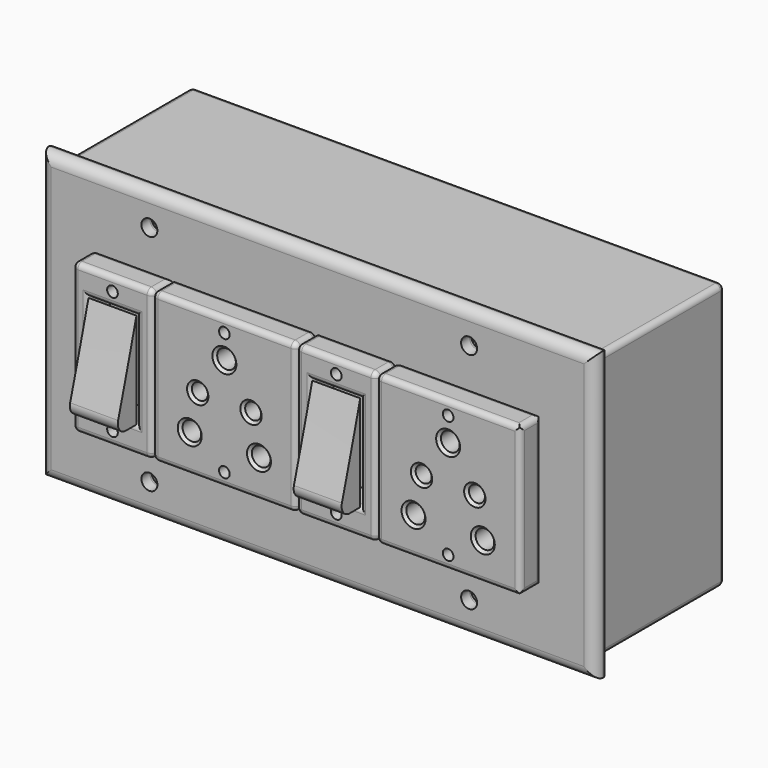
from build123d import *

# Parameters (mm, degrees)
F0_W           = 10
F0_H           = 5
F1_DEPTH       = 3
F2_T           = -0.5
F3_W           = 10.4
F3_H           = 5.4
F3_W_2         = 10
F3_H_2         = 5
F3_W_3         = 9
F3_H_3         = 4
F4_DEPTH       = 0.3
F5_W           = 1.5
F5_H           = 2.8
F5_W_2         = 0.9
F5_H_2         = 1.8
F6_DEPTH       = 0.5
F5_W_3         = 2.7
F5_R           = 0.175
F5_R_2         = 0.15
F7_DEPTH       = 0.5
F9_DEPTH       = 0.9
F10_R          = 0.1
F11_SIZE       = 0.05
F12_R          = 0.1
F13_R          = 0.2
F15_D          = 0.2
F15_DEPTH      = 0.5
F15_TIP        = 0.0600860619
F15_2_D        = 0.2
F15_2_DEPTH    = 0.5
F15_2_TIP      = 0.0600860619
F15_3_D        = 0.2
F15_3_DEPTH    = 0.5
F15_3_TIP      = 0.0600860619
F17_D          = 0.3
F17_DEPTH      = 0.5
F17_TIP        = 0.0901290929
F17_2_D        = 0.3
F17_2_DEPTH    = 0.5
F17_2_TIP      = 0.0901290929
F22_T1_DEPTH   = 2.6
F22_S5_W       = 0.1
F22_S5_H       = 0.1
F22_T6_DEPTH   = 0.1
F22_S11_W      = 0.1
F22_S11_H      = 0.1
F22_T12_DEPTH  = 0.1
F22_2_T1_DEPTH = 3.1
F23_R          = 0.09999
F23_2_R        = 0.09999


# Not quite as in the source:
# - a fillet or chamfer that OpenCascade refuses, or shapes differently, is made with other operations: its cross-section is extruded or revolved along the edge and cut away or added
# - a fillet or chamfer is up to 0.001 mm smaller than in the source, because OpenCascade refuses the exact size


with BuildPart() as f1:
    # F0 (on Front) → F1 (new body)
    with BuildSketch(Plane.XZ):
        Rectangle(F0_W, F0_H)
    extrude(amount=F1_DEPTH)

    # F2
    f2_openings = [f1.faces().sort_by_distance(p)[0] for p in [
        (0, -3, 0),
    ]]
    offset(amount=F2_T, openings=f2_openings)

    # F17
    with Locations(Plane.XZ.offset(3.3)):
        with Locations((-3.1569213606, 2.1), (2.8430786394, 2.1), (-3.1569213606, -2.1), (2.8430786394, -2.1)):
            Hole(F17_D / 2, depth=F17_DEPTH)
            with Locations((0, 0, -(F17_DEPTH + F17_TIP / 2))):  # 118° drill point
                Cone(0, F17_D / 2, F17_TIP, mode=Mode.SUBTRACT)

    # F23 (radius 0.1 in the source; OpenCascade refuses exactly that, so slightly less here)
    f23_edges = [f1.edges().sort_by_distance(p)[0] for p in [
        (5, -1.5, -2.5),
        (5, -1.5, 2.5),
        (5, 0, 0),
        (5, -3, 0),
        (-5, -1.5, 2.5),
        (0, 0, 2.5),
        (0, -3, 2.5),
        (0, 0, -2.5),
        (-5, 0, 0),
        (-5, -1.5, -2.5),
        (-5, -3, 0),
    ]]
    fillet(f23_edges, radius=F23_R)


with BuildPart() as f4:
    # F3 (on face) → F4 (new body)
    with BuildSketch(Plane.XZ.offset(3)):
        Rectangle(F3_W, F3_H)
        Rectangle(F3_W_2, F3_H_2, mode=Mode.SUBTRACT)
        Rectangle(F3_W_2, F3_H_2)
        Rectangle(F3_W_3, F3_H_3, mode=Mode.SUBTRACT)
        Rectangle(F3_W_3, F3_H_3)
    extrude(amount=F4_DEPTH)

    # F13
    f13_edges = [f4.edges().sort_by_distance(p)[0] for p in [
        (0, -3.3, -2.7),
        (5.2, -3.3, 0),
        (0, -3.3, 2.7),
        (-5.2, -3.3, 0),
    ]]
    fillet(f13_edges, radius=F13_R)

    # F15
    with Locations(Plane.XZ.offset(3.8)):
        with Locations((-3.45, 1.15), (-1.35, 1.15), (-3.45, -1.15), (-1.35, -1.15)):
            Hole(F15_D / 2, depth=F15_DEPTH)
            with Locations((0, 0, -(F15_DEPTH + F15_TIP / 2))):  # 118° drill point
                Cone(0, F15_D / 2, F15_TIP, mode=Mode.SUBTRACT)

    # F17#2
    with Locations(Plane.XZ.offset(3.3)):
        with Locations((-3.1569213606, 2.1), (2.8430786394, 2.1), (-3.1569213606, -2.1), (2.8430786394, -2.1)):
            Hole(F17_2_D / 2, depth=F17_2_DEPTH)
            with Locations((0, 0, -(F17_2_DEPTH + F17_2_TIP / 2))):  # 118° drill point
                Cone(0, F17_2_D / 2, F17_2_TIP, mode=Mode.SUBTRACT)

    # F23#2 (radius 0.1 in the source; OpenCascade refuses exactly that, so slightly less here)
    f23_2_edges = [f4.edges().sort_by_distance(p)[0] for p in [
        (0, -3, -2.7),
        (-5.2, -3, 0),
        (5.2, -3, 0),
        (0, -3, 2.7),
        (-3.306921, -3, -2.1),
        (2.693079, -3, -2.1),
        (-3.306921, -3, 2.1),
        (2.693079, -3, 2.1),
    ]]
    fillet(f23_2_edges, radius=F23_2_R)


with BuildPart() as f6:
    # F5 (on face) → F6 (new body)
    with BuildSketch(Plane.XZ.offset(3.3)):
        with Locations((-3.45, 0)):
            Rectangle(F5_W, F5_H)
        with Locations((-3.45, 0)):
            Rectangle(F5_W_2, F5_H_2, mode=Mode.SUBTRACT)
    extrude(amount=F6_DEPTH)

    # F10
    f10_edges = [f6.edges().sort_by_distance(p)[0] for p in [
        (-3.45, -3.8, -1.4),
        (-2.7, -3.8, 0),
        (-3.45, -3.8, 1.4),
        (-4.2, -3.8, 0),
        (-3, -3.8, 0),
        (-3.45, -3.8, -0.9),
        (-3.9, -3.8, 0),
        (-3.45, -3.8, 0.9),
        (-4.2, -3.55, 1.4),
        (-4.2, -3.55, -1.4),
        (-4.2, -3.3, 0),
        (-3.45, -3.3, 1.4),
        (-3.45, -3.3, -1.4),
        (-2.7, -3.55, 1.4),
        (-2.7, -3.55, -1.4),
    ]]
    fillet(f10_edges, radius=F10_R)

    # F15#2
    with Locations(Plane.XZ.offset(3.8)):
        with Locations((-3.45, 1.15), (-1.35, 1.15), (-3.45, -1.15), (-1.35, -1.15)):
            Hole(F15_2_D / 2, depth=F15_2_DEPTH)
            with Locations((0, 0, -(F15_2_DEPTH + F15_2_TIP / 2))):  # 118° drill point
                Cone(0, F15_2_D / 2, F15_2_TIP, mode=Mode.SUBTRACT)


with BuildPart() as f7:
    # F5 (on face) → F7 (new body)
    with BuildSketch(Plane.XZ.offset(3.3)):
        with Locations((-1.35, 0)):
            Rectangle(F5_W_3, F5_H)
        with Locations((-2, -0.7)):
            Circle(F5_R, mode=Mode.SUBTRACT)
        with Locations((-0.7, -0.7)):
            Circle(F5_R, mode=Mode.SUBTRACT)
        with Locations((-1.85, 0)):
            Circle(F5_R_2, mode=Mode.SUBTRACT)
        with Locations((-0.85, 0)):
            Circle(F5_R_2, mode=Mode.SUBTRACT)
        with Locations((-1.35, 0.7)):
            Circle(F5_R, mode=Mode.SUBTRACT)
    extrude(amount=F7_DEPTH)

    # F11
    f11_edges = [f7.edges().sort_by_distance(p)[0] for p in [
        (-1.525, -3.8, 0.7),
        (-2, -3.8, 0),
        (-1, -3.8, 0),
        (-2.175, -3.8, -0.7),
        (-0.875, -3.8, -0.7),
    ]]
    chamfer(f11_edges, length=F11_SIZE)

    # F12
    f12_edges = [f7.edges().sort_by_distance(p)[0] for p in [
        (0, -3.55, 1.4),
        (-2.7, -3.55, 1.4),
        (-1.35, -3.3, 1.4),
        (-1.35, -3.8, 1.4),
        (0, -3.55, -1.4),
        (0, -3.3, 0),
        (0, -3.8, 0),
        (-2.7, -3.55, -1.4),
        (-1.35, -3.3, -1.4),
        (-1.35, -3.8, -1.4),
    ]]
    fillet(f12_edges, radius=F12_R)

    # F15#3
    with Locations(Plane.XZ.offset(3.8)):
        with Locations((-3.45, 1.15), (-1.35, 1.15), (-3.45, -1.15), (-1.35, -1.15)):
            Hole(F15_3_D / 2, depth=F15_3_DEPTH)
            with Locations((0, 0, -(F15_3_DEPTH + F15_3_TIP / 2))):  # 118° drill point
                Cone(0, F15_3_D / 2, F15_3_TIP, mode=Mode.SUBTRACT)


with BuildPart() as f9:
    # F8 (on face) → F9 (new body, through all)
    with BuildSketch(Plane.YZ.offset(-3.9)):
        with BuildLine():
            Line((-4.0475652224, -0.9), (-3.8, -0.9))
            Line((-3.8, -0.9), (-3.8, 0.9))
            ThreePointArc((-3.8, 0.9), (-4.0115602658, 0.1201773265), (-4.230279809, -0.6576677157))
            ThreePointArc((-4.230279809, -0.6576677157), (-4.1993130034, -0.8243672998), (-4.0475652224, -0.9))
        make_face()
    extrude(amount=F9_DEPTH)


with BuildPart() as f19_1:
    # F19: instance of F6
    add(f6.part.mirror(Plane.YZ.offset(-1.35)))


with BuildPart() as f19_2:
    # F19: instance of F9
    add(f9.part.mirror(Plane.YZ.offset(-1.35)))


with BuildPart() as f21_1:
    # F21: instance of F7
    add(f7.part.mirror(Plane.YZ.offset(0.75)))

    # F22#2: fillet of radius 0.1 on 4 edges, made by hand

    # F22_2_s2 → F22_2_t1 (cut)
    with BuildSketch(Plane.XY.offset(-1.55)):
        with BuildLine():
            ThreePointArc((4.1, -3.3), (4.1707106781, -3.3292893219), (4.2, -3.4))
            Line((4.2, -3.4), (4.2, -3.3))
            Line((4.2, -3.3), (4.1, -3.3))
        make_face()
        with BuildLine():
            ThreePointArc((4.2, -3.7), (4.1707106781, -3.7707106781), (4.1, -3.8))
            Line((4.1, -3.8), (4.2, -3.8))
            Line((4.2, -3.8), (4.2, -3.7))
        make_face()
    extrude(amount=F22_2_T1_DEPTH, mode=Mode.SUBTRACT)


with BuildPart() as f7_1:
    add(f7.part)

    # F22: fillet of radius 0.1 on 1 edges, made by hand

    # F22_s2 → F22_t1 (cut)
    with BuildSketch(Plane.XY.offset(-1.3)):
        with BuildLine():
            ThreePointArc((-2.7, -3.7), (-2.6707106781, -3.7707106781), (-2.6, -3.8))
            Line((-2.6, -3.8), (-2.7, -3.8))
            Line((-2.7, -3.8), (-2.7, -3.7))
        make_face()
    extrude(amount=F22_T1_DEPTH, mode=Mode.SUBTRACT)


with BuildPart() as f22_tool4:
    # F22_s5 → F22_t6 (new body)
    with BuildSketch(Plane.YZ.offset(-2.6)):
        with Locations((-3.75, 1.35)):
            Rectangle(F22_S5_W, F22_S5_H)
    extrude(amount=-F22_T6_DEPTH)

    # F22_s7 → F22_t8 (revolve, cut)
    with BuildSketch(Plane(origin=(-2.6, -3.7, 1.3), x_dir=(0, 0.7071067812, -0.7071067812), z_dir=(0, 0.7071067812, 0.7071067812))):
        with BuildLine():
            ThreePointArc((0, -0.1), (0.1, 0), (0, 0.1))
            Line((0, 0.1), (0, -0.1))
        make_face()
    revolve(axis=Axis((-2.6, -3.7, 1.3), (-1, 0, 0)), mode=Mode.SUBTRACT)


with BuildPart() as f7_2:
    add(f7_1.part)

    # F22_t3: cut F22_tool4
    add(f22_tool4.part, mode=Mode.SUBTRACT)


with BuildPart() as f22_tool10:
    # F22_s11 → F22_t12 (new body)
    with BuildSketch(Plane.YZ.offset(-2.6)):
        with Locations((-3.75, -1.35)):
            Rectangle(F22_S11_W, F22_S11_H)
    extrude(amount=-F22_T12_DEPTH)

    # F22_s13 → F22_t14 (revolve, cut)
    with BuildSketch(Plane(origin=(-2.6, -3.7, -1.3), x_dir=(0, 0.7071067812, 0.7071067812), z_dir=(0, -0.7071067812, 0.7071067812))):
        with BuildLine():
            ThreePointArc((0, -0.1), (0.1, 0), (0, 0.1))
            Line((0, 0.1), (0, -0.1))
        make_face()
    revolve(axis=Axis((-2.6, -3.7, -1.3), (-1, 0, 0)), mode=Mode.SUBTRACT)


with BuildPart() as f7_3:
    add(f7_2.part)

    # F22_t9: cut F22_tool10
    add(f22_tool10.part, mode=Mode.SUBTRACT)


solid = Compound([f1.part, f4.part, f6.part, f9.part, f19_1.part, f19_2.part, f21_1.part, f7_3.part])
